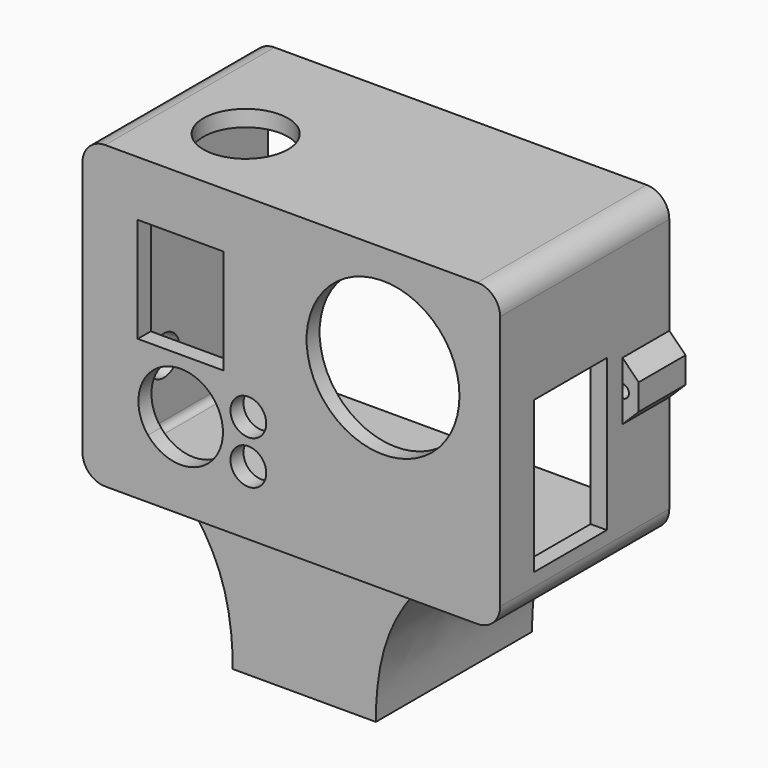
from build123d import *

# Parameters (mm, degrees)
F1_DEPTH  = 30
F0_R      = 2.75
F0_W      = 13.2
F0_H      = 16.1
F0_R_2    = 11.75
F2_DEPTH  = 2.5
F3_R      = 6.5
F4_DEPTH  = 2.5
F5_R      = 3
F6_DEPTH  = 2.5
F7_W      = 14
F7_H      = 23.3
F8_DEPTH  = 2.5
F5_W      = 9
F5_H      = 9
F9_DEPTH  = 2.5
F7_W_2    = 9
F7_H_2    = 9
F10_DEPTH = 2.5
F11_SIZE  = 2.49999
F12_R     = 1
F13_DEPTH = 9


# Not quite as in the source:
# - a fillet or chamfer is up to 0.001 mm smaller than in the source, because OpenCascade refuses the exact size


with BuildPart() as f1:
    # F0 (on Front) → F1 (new body)
    with BuildSketch(Plane.XZ):
        with BuildLine():
            Line((-28.6, 20.6), (28.6, 20.6))
            ThreePointArc((28.6, 20.6), (29.3071067812, 20.3071067812), (29.6, 19.6))
            Line((29.6, 19.6), (29.6, -19.6))
            ThreePointArc((29.6, -19.6), (29.3071067812, -20.3071067812), (28.6, -20.6))
            Line((28.6, -20.6), (19.2463447419, -20.6))
            add(Edge.make_bspline(
                [(19.2463447419, -20.6), (18.6700440776, -21.4257741259), (18.043869698, -22.2429184725), (17.402758481, -23.1)],
                knots=[11.0100107819, 11.0100107819, 11.0100107819, 11.0100107819, 14.8362531821, 14.8362531821, 14.8362531821, 14.8362531821], degree=3))
            Line((17.402758481, -23.1), (28.6, -23.1))
            ThreePointArc((28.6, -23.1), (31.0748737342, -22.0748737342), (32.1, -19.6))
            Line((32.1, -19.6), (32.1, 19.6))
            ThreePointArc((32.1, 19.6), (31.0748737342, 22.0748737342), (28.6, 23.1))
            Line((28.6, 23.1), (-28.6, 23.1))
            ThreePointArc((-28.6, 23.1), (-31.0748737342, 22.0748737342), (-32.1, 19.6))
            Line((-32.1, 19.6), (-32.1, -19.6))
            ThreePointArc((-32.1, -19.6), (-31.0748737342, -22.0748737342), (-28.6, -23.1))
            Line((-28.6, -23.1), (-17.402758481, -23.1))
            add(Edge.make_bspline(
                [(-19.2463447419, -20.6), (-18.6700440776, -21.4257741259), (-18.043869698, -22.2429184725), (-17.402758481, -23.1)],
                knots=[11.0100107819, 11.0100107819, 11.0100107819, 11.0100107819, 14.8362531821, 14.8362531821, 14.8362531821, 14.8362531821], degree=3))
            Line((-19.2463447419, -20.6), (-28.6, -20.6))
            ThreePointArc((-28.6, -20.6), (-29.3071067812, -20.3071067812), (-29.6, -19.6))
            Line((-29.6, -19.6), (-29.6, 19.6))
            ThreePointArc((-29.6, 19.6), (-29.3071067812, 20.3071067812), (-28.6, 20.6))
        make_face()
        with BuildLine():
            add(Edge.make_bspline(
                [(19.2463447419, -20.6), (18.6700440776, -21.4257741259), (18.043869698, -22.2429184725), (17.402758481, -23.1)],
                knots=[11.0100107819, 11.0100107819, 11.0100107819, 11.0100107819, 14.8362531821, 14.8362531821, 14.8362531821, 14.8362531821], degree=3))
            Line((19.2463447419, -20.6), (-19.2463447419, -20.6))
            add(Edge.make_bspline(
                [(-19.2463447419, -20.6), (-18.6700440776, -21.4257741259), (-18.043869698, -22.2429184725), (-17.402758481, -23.1)],
                knots=[11.0100107819, 11.0100107819, 11.0100107819, 11.0100107819, 14.8362531821, 14.8362531821, 14.8362531821, 14.8362531821], degree=3))
            Line((-17.402758481, -23.1), (17.402758481, -23.1))
        make_face()
        with BuildLine():
            add(Edge.make_bspline(
                [(17.402758481, -23.1), (14.3686514172, -27.1562028058), (11, -32.1068893696), (11, -43.1)],
                knots=[14.8362531821, 14.8362531821, 14.8362531821, 14.8362531821, 32.9442331828, 32.9442331828, 32.9442331828, 32.9442331828], degree=3))
            Line((17.402758481, -23.1), (-17.402758481, -23.1))
            add(Edge.make_bspline(
                [(-17.402758481, -23.1), (-14.3686514172, -27.1562028058), (-11, -32.1068893696), (-11, -43.1)],
                knots=[14.8362531821, 14.8362531821, 14.8362531821, 14.8362531821, 32.9442331828, 32.9442331828, 32.9442331828, 32.9442331828], degree=3))
            Line((-11, -43.1), (11, -43.1))
        make_face()
    extrude(amount=-F1_DEPTH)

    # F0 (on Front) → F2 (join)
    with BuildSketch(Plane.XZ):
        with BuildLine():
            Line((-28.6, 20.6), (28.6, 20.6))
            ThreePointArc((28.6, 20.6), (29.3071067812, 20.3071067812), (29.6, 19.6))
            Line((29.6, 19.6), (29.6, -19.6))
            ThreePointArc((29.6, -19.6), (29.3071067812, -20.3071067812), (28.6, -20.6))
            Line((28.6, -20.6), (19.2463447419, -20.6))
            add(Edge.make_bspline(
                [(19.2463447419, -20.6), (18.6700440776, -21.4257741259), (18.043869698, -22.2429184725), (17.402758481, -23.1)],
                knots=[11.0100107819, 11.0100107819, 11.0100107819, 11.0100107819, 14.8362531821, 14.8362531821, 14.8362531821, 14.8362531821], degree=3))
            Line((17.402758481, -23.1), (28.6, -23.1))
            ThreePointArc((28.6, -23.1), (31.0748737342, -22.0748737342), (32.1, -19.6))
            Line((32.1, -19.6), (32.1, 19.6))
            ThreePointArc((32.1, 19.6), (31.0748737342, 22.0748737342), (28.6, 23.1))
            Line((28.6, 23.1), (-28.6, 23.1))
            ThreePointArc((-28.6, 23.1), (-31.0748737342, 22.0748737342), (-32.1, 19.6))
            Line((-32.1, 19.6), (-32.1, -19.6))
            ThreePointArc((-32.1, -19.6), (-31.0748737342, -22.0748737342), (-28.6, -23.1))
            Line((-28.6, -23.1), (-17.402758481, -23.1))
            add(Edge.make_bspline(
                [(-19.2463447419, -20.6), (-18.6700440776, -21.4257741259), (-18.043869698, -22.2429184725), (-17.402758481, -23.1)],
                knots=[11.0100107819, 11.0100107819, 11.0100107819, 11.0100107819, 14.8362531821, 14.8362531821, 14.8362531821, 14.8362531821], degree=3))
            Line((-19.2463447419, -20.6), (-28.6, -20.6))
            ThreePointArc((-28.6, -20.6), (-29.3071067812, -20.3071067812), (-29.6, -19.6))
            Line((-29.6, -19.6), (-29.6, 19.6))
            ThreePointArc((-29.6, 19.6), (-29.3071067812, 20.3071067812), (-28.6, 20.6))
        make_face()
        with BuildLine():
            ThreePointArc((29.6, 19.6), (29.3071067812, 20.3071067812), (28.6, 20.6))
            Line((28.6, 20.6), (-28.6, 20.6))
            ThreePointArc((-28.6, 20.6), (-29.3071067812, 20.3071067812), (-29.6, 19.6))
            Line((-29.6, 19.6), (-29.6, -19.6))
            ThreePointArc((-29.6, -19.6), (-29.3071067812, -20.3071067812), (-28.6, -20.6))
            Line((-28.6, -20.6), (-19.2463447419, -20.6))
            Line((-19.2463447419, -20.6), (19.2463447419, -20.6))
            Line((19.2463447419, -20.6), (28.6, -20.6))
            ThreePointArc((28.6, -20.6), (29.3071067812, -20.3071067812), (29.6, -19.6))
            Line((29.6, -19.6), (29.6, 19.6))
        make_face()
        with Locations((-6.6, -13.25)):
            Circle(F0_R, mode=Mode.SUBTRACT)
        with BuildLine():
            ThreePointArc((-10.5, -9.9), (-14.8124838728, -16.0208474244), (-22.027622521, -14.019831524))
            ThreePointArc((-22.027622521, -14.019831524), (-19.1875161272, -3.7791525756), (-10.5, -9.9))
        make_face(mode=Mode.SUBTRACT)
        with Locations((-17, 6.55)):
            Rectangle(F0_W, F0_H, mode=Mode.SUBTRACT)
        with Locations((-6.6, -6.55)):
            Circle(F0_R, mode=Mode.SUBTRACT)
        with Locations((14.1, 6.85)):
            Circle(F0_R_2, mode=Mode.SUBTRACT)
        with BuildLine():
            add(Edge.make_bspline(
                [(19.2463447419, -20.6), (18.6700440776, -21.4257741259), (18.043869698, -22.2429184725), (17.402758481, -23.1)],
                knots=[11.0100107819, 11.0100107819, 11.0100107819, 11.0100107819, 14.8362531821, 14.8362531821, 14.8362531821, 14.8362531821], degree=3))
            Line((19.2463447419, -20.6), (-19.2463447419, -20.6))
            add(Edge.make_bspline(
                [(-19.2463447419, -20.6), (-18.6700440776, -21.4257741259), (-18.043869698, -22.2429184725), (-17.402758481, -23.1)],
                knots=[11.0100107819, 11.0100107819, 11.0100107819, 11.0100107819, 14.8362531821, 14.8362531821, 14.8362531821, 14.8362531821], degree=3))
            Line((-17.402758481, -23.1), (17.402758481, -23.1))
        make_face()
    extrude(amount=F2_DEPTH)

    # F3 (on face) → F4 (cut, through all)
    with BuildSketch(Plane.XY.offset(23.1)):
        with Locations((-17.25, 10.3)):
            Circle(F3_R)
    extrude(amount=-F4_DEPTH, mode=Mode.SUBTRACT)

    # F5 (on face) → F6 (cut, through all)
    with BuildSketch(Plane(origin=(-32.1, 0, 0), x_dir=(0, -1, 0), z_dir=(-1, 0, 0))):
        with Locations((-10, -10.8)):
            Circle(F5_R)
    extrude(amount=-F6_DEPTH, mode=Mode.SUBTRACT)

    # F7 (on face) → F8 (cut, through all)
    with BuildSketch(Plane.YZ.offset(32.1)):
        with Locations((11, -5.95)):
            Rectangle(F7_W, F7_H)
    extrude(amount=-F8_DEPTH, mode=Mode.SUBTRACT)

    # F5 (on face) → F9 (join)
    with BuildSketch(Plane(origin=(-32.1, 0, 0), x_dir=(0, -1, 0), z_dir=(-1, 0, 0))):
        with Locations((-25.5, 0)):
            Rectangle(F5_W, F5_H)
    extrude(amount=F9_DEPTH)

    # F7 (on face) → F10 (join)
    with BuildSketch(Plane.YZ.offset(32.1)):
        with Locations((25.5, 0)):
            Rectangle(F7_W_2, F7_H_2)
    extrude(amount=F10_DEPTH)

    # F11 (size 2.5 in the source; OpenCascade refuses exactly that, so slightly less here)
    f11_edges = [f1.edges().sort_by_distance(p)[0] for p in [
        (-34.6, 25.5, -4.5),
        (-34.6, 25.5, 4.5),
        (34.6, 25.5, 4.5),
        (34.6, 25.5, -4.5),
    ]]
    chamfer(f11_edges, length=F11_SIZE)

    # F12 (on face) → F13 (cut)
    with BuildSketch(Plane(origin=(0, 30, 0), x_dir=(-1, 0, 0), z_dir=(0, 1, 0))):
        with Locations((-32.1, 0)):
            Circle(F12_R)
        with Locations((32.1, 0)):
            Circle(F12_R)
    extrude(amount=-F13_DEPTH, mode=Mode.SUBTRACT)


solid = f1.part
